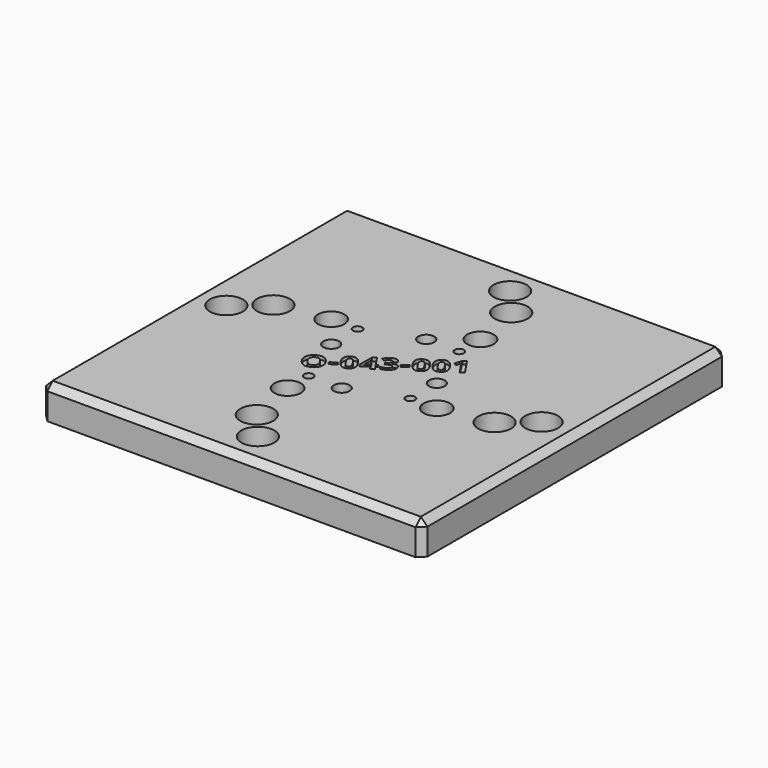
from build123d import *

# Parameters (mm, degrees)
F0_R         = 5
F0_R_2       = 4
F0_R_3       = 1.405
F0_R_4       = 2.395
F1_DEPTH     = 10
F2_TEXT_SIZE = 8.3835472884
F3_DEPTH     = 1
F4_SIZE      = 2


# Not quite as in the source:
# - Text() gives the source's letters only with a copy of the font that has no kerning and outlines rounded to 1/6400 em; it was checked with that copy


with BuildPart() as f1:
    # F0 (on Top) → F1 (new body)
    with BuildSketch(Plane.XY):
        Polygon((-57.75, -57.75), (-21, -57.75), (10, -57.75), (57.75, -57.75), (57.75, -21), (57.75, 10), (57.75, 57.75), (21, 57.75), (-10, 57.75), (-57.75, 57.75), align=None)
        with Locations((-7.1482573643, -39.2255799484)):
            Circle(F0_R, mode=Mode.SUBTRACT)
        with Locations((-10, -24)):
            Circle(F0_R_2, mode=Mode.SUBTRACT)
        with Locations((-10, -16)):
            Circle(F0_R_3, mode=Mode.SUBTRACT)
        with Locations((0, -47.75)):
            Circle(F0_R, mode=Mode.SUBTRACT)
        with Locations((0, -16)):
            Circle(F0_R_4, mode=Mode.SUBTRACT)
        with Locations((16, -10)):
            Circle(F0_R_3, mode=Mode.SUBTRACT)
        with Locations((24, -10)):
            Circle(F0_R_2, mode=Mode.SUBTRACT)
        with Locations((39.2255799484, -7.1482573643)):
            Circle(F0_R, mode=Mode.SUBTRACT)
        with Locations((-47.75, 0)):
            Circle(F0_R, mode=Mode.SUBTRACT)
        with Locations((-39.2255799484, 7.1482573643)):
            Circle(F0_R, mode=Mode.SUBTRACT)
        with Locations((-16, 0)):
            Circle(F0_R_4, mode=Mode.SUBTRACT)
        with Locations((-24, 10)):
            Circle(F0_R_2, mode=Mode.SUBTRACT)
        with Locations((-16, 10)):
            Circle(F0_R_3, mode=Mode.SUBTRACT)
        with Locations((16, 0)):
            Circle(F0_R_4, mode=Mode.SUBTRACT)
        with Locations((0, 16)):
            Circle(F0_R_4, mode=Mode.SUBTRACT)
        with Locations((10, 16)):
            Circle(F0_R_3, mode=Mode.SUBTRACT)
        with Locations((10, 24)):
            Circle(F0_R_2, mode=Mode.SUBTRACT)
        with Locations((47.75, 0)):
            Circle(F0_R, mode=Mode.SUBTRACT)
        with Locations((7.1482573643, 39.2255799484)):
            Circle(F0_R, mode=Mode.SUBTRACT)
        with Locations((0, 47.75)):
            Circle(F0_R, mode=Mode.SUBTRACT)
    extrude(amount=F1_DEPTH)

    # F2 (on face) → F3 (cut)
    with BuildSketch(Plane.XY.offset(10)):
        with Locations(Location((-14.8930641972, -13.685957319), (0, 0, 34))):
            Text('O-043-001', F2_TEXT_SIZE, font='Open Sans', font_style=FontStyle.BOLD, text_align=(TextAlign.LEFT, TextAlign.BOTTOM))
    extrude(amount=-F3_DEPTH, mode=Mode.SUBTRACT)

    # F4
    f4_edges = [f1.edges().sort_by_distance(p)[0] for p in [
        (-57.75, -57.75, 5),
        (57.75, -57.75, 5),
        (57.75, 57.75, 5),
        (-57.75, 57.75, 5),
        (0, 57.75, 10),
        (57.75, 0, 10),
        (0, -57.75, 10),
        (-57.75, 0, 10),
    ]]
    chamfer(f4_edges, length=F4_SIZE)


solid = f1.part
